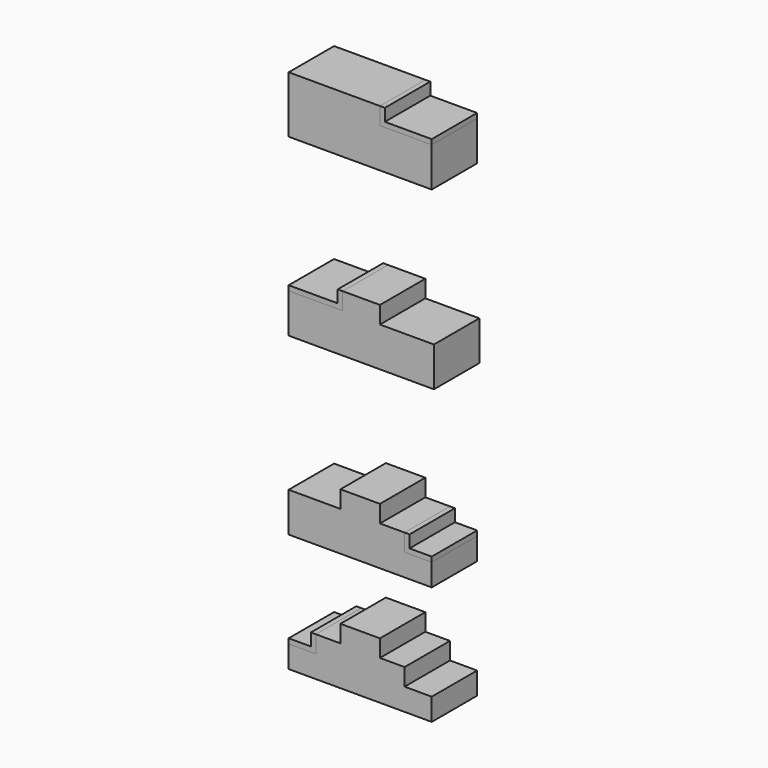
from build123d import *

# Parameters (mm, degrees)
F4_DEPTH = 23
F5_DEPTH = 23


# Not quite as in the source:
# - a feature names something its author has since deleted; it is built from what else it names


with BuildPart() as f4:
    # F2 (on Front) → F4 (new body)
    with BuildSketch(Plane.XZ):
        Polygon((67, 181), (51.8985245079, 181), (51.8985245079, 174), (30, 174), (30, 158), (88.8985245079, 158), (88.8985245079, 174), (67, 174), align=None)
    extrude(amount=F4_DEPTH)


with BuildPart() as f4b:
    # F1 (on Front) → F4, piece 2 (new body)
    with BuildSketch(Plane.XZ):
        Polygon((67, 252), (30, 252), (30, 229), (88, 229), (88, 245), (67, 245), align=None)
    extrude(amount=F4_DEPTH)


with BuildPart() as f4c:
    # F3 (on Front) → F4, piece 3 (new body)
    with BuildSketch(Plane.XZ):
        Polygon((67, 110), (51, 110), (51, 103), (41, 103), (30, 103), (30, 96), (30, 87), (88, 87), (88, 96), (77, 96), (77, 103), (67, 103), align=None)
    extrude(amount=F4_DEPTH)


with BuildPart() as f4d:
    # F3 (on Front) → F4, piece 4 (new body)
    with BuildSketch(Plane.XZ):
        Polygon((51, 55), (41, 55), (41, 48), (30, 48), (30, 39), (88, 39), (88, 48), (77, 48), (77, 55), (67, 55), (67, 62), (51, 62), align=None)
    extrude(amount=F4_DEPTH)


with BuildPart() as f5:
    # F2 (on Front) → F5 (new body)
    with BuildSketch(Plane.XZ):
        Polygon((51.8985245079, 181), (49.8985245079, 181), (49.8985245079, 176), (30, 176), (30, 174), (51.8985245079, 174), align=None)
    extrude(amount=F5_DEPTH)


with BuildPart() as f5b:
    # F3 (on Front) → F5, piece 2 (new body)
    with BuildSketch(Plane.XZ):
        Polygon((79, 103), (77, 103), (77, 96), (88, 96), (88, 98), (79, 98), align=None)
    extrude(amount=F5_DEPTH)


with BuildPart() as f5c:
    # F3 (on Front) → F5, piece 3 (new body)
    with BuildSketch(Plane.XZ):
        Polygon((41, 48), (41, 55), (39, 55), (39, 50), (30, 50), (30, 48), align=None)
    extrude(amount=F5_DEPTH)


with BuildPart() as f5d:
    # F1 (on Front) → F5, piece 4 (new body)
    with BuildSketch(Plane.XZ):
        Polygon((69, 252), (67, 252), (67, 245), (88, 245), (88, 247), (69, 247), align=None)
    extrude(amount=F5_DEPTH)


solid = Compound([f4.part, f4b.part, f4c.part, f4d.part, f5.part, f5b.part, f5c.part, f5d.part])
